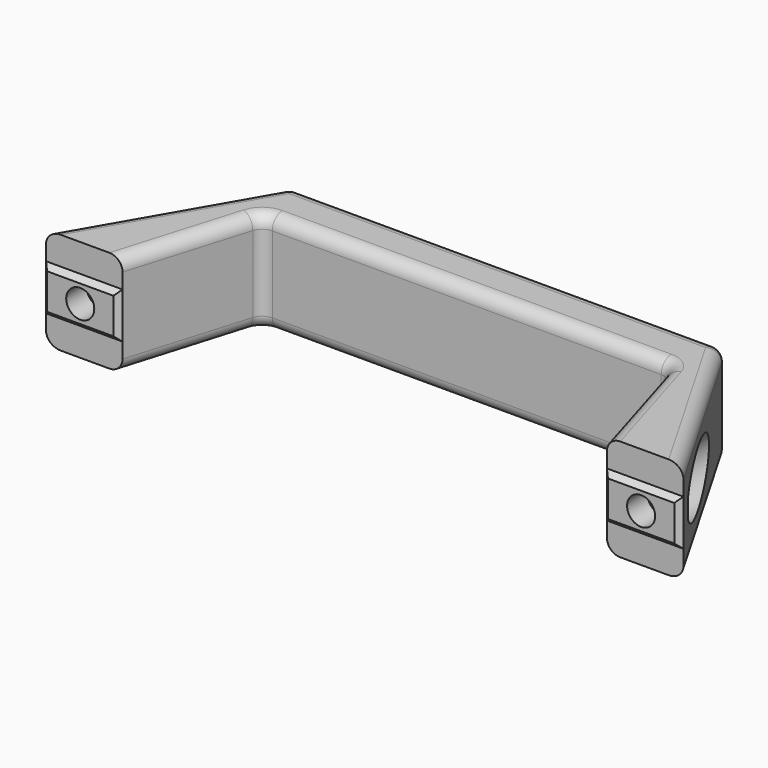
from build123d import *

# Parameters (mm, degrees)
F1_DEPTH = 20
F2_W     = 15
F2_H     = 9
F3_DEPTH = 1
F4_R     = 2.75
F5_DEPTH = 36.001
F6_R     = 5.5
F7_DEPTH = 31
F8_F1_R  = 2.5
F8_F2_R  = 2.5
F9_SIZE  = 0.99999


# Not quite as in the source:
# - a fillet or chamfer is up to 0.001 mm smaller than in the source, because OpenCascade refuses the exact size


with BuildPart() as f1:
    # F0 (on Top) → F1 (new body)
    with BuildSketch(Plane.XY):
        Polygon((20.2072594216, 35), (0, 0), (15, 0), (22.5, 25), (102.5, 25), (110, 0), (125, 0), (104.7927405784, 35), align=None)
    extrude(amount=F1_DEPTH)

    # F2 (on face) → F3 (join)
    with BuildSketch(Plane.XZ):
        with Locations((7.5, 10)):
            Rectangle(F2_W, F2_H)
        with Locations((117.5, 10)):
            Rectangle(F2_W, F2_H)
    extrude(amount=F3_DEPTH)

    # F4 (on face) → F5 (cut, through all)
    with BuildSketch(Plane.XZ.offset(1)):
        with Locations((7.5, 10)):
            Circle(F4_R)
        with Locations((117.5, 10)):
            Circle(F4_R)
    extrude(amount=-F5_DEPTH, mode=Mode.SUBTRACT)

    # F6 (on face) → F7 (cut)
    with BuildSketch(Plane(origin=(0, 35, 0), x_dir=(-1, 0, 0), z_dir=(0, 1, 0))):
        with Locations((-117.5, 10)):
            Circle(F6_R)
        with Locations((-7.5, 10)):
            Circle(F6_R)
    extrude(amount=-F7_DEPTH, mode=Mode.SUBTRACT)

    # F8: fillet of radius 2.5 on 12 edges, made by hand

    # F8_f1
    f8_f1_edges = [f1.edges().sort_by_distance(p)[0] for p in [
        (22.5, 25, 10),
        (102.5, 25, 10),
    ]]
    fillet(f8_f1_edges, radius=F8_F1_R)

    # F8_f2
    f8_f2_edges = [f1.edges().sort_by_distance(p)[0] for p in [
        (62.5, 25, 0),
        (62.5, 25, 20),
        (104.7927405784, 35, 10),
        (20.2072594216, 35, 10),
        (62.5, 35, 0),
        (62.5, 35, 20),
        (114.8963702892, 17.5, 20),
        (114.8963702892, 17.5, 0),
        (10.1036297108, 17.5, 20),
        (10.1036297108, 17.5, 0),
        (22.8677503031, 24.5057323207, 20),
        (102.1322496969, 24.5057323207, 20),
        (22.8677503031, 24.5057323207, 0),
        (102.1322496969, 24.5057323207, 0),
    ]]
    fillet(f8_f2_edges, radius=F8_F2_R)

    # F9 (size 1 in the source; OpenCascade refuses exactly that, so slightly less here)
    f9_edges = [f1.edges().sort_by_distance(p)[0] for p in [
        (7.5, -1, 14.5),
        (0, -1, 10),
        (7.5, -1, 5.5),
        (15, -1, 10),
        (117.5, -1, 14.5),
        (110, -1, 10),
        (117.5, -1, 5.5),
        (125, -1, 10),
    ]]
    chamfer(f9_edges, length=F9_SIZE)


solid = f1.part
